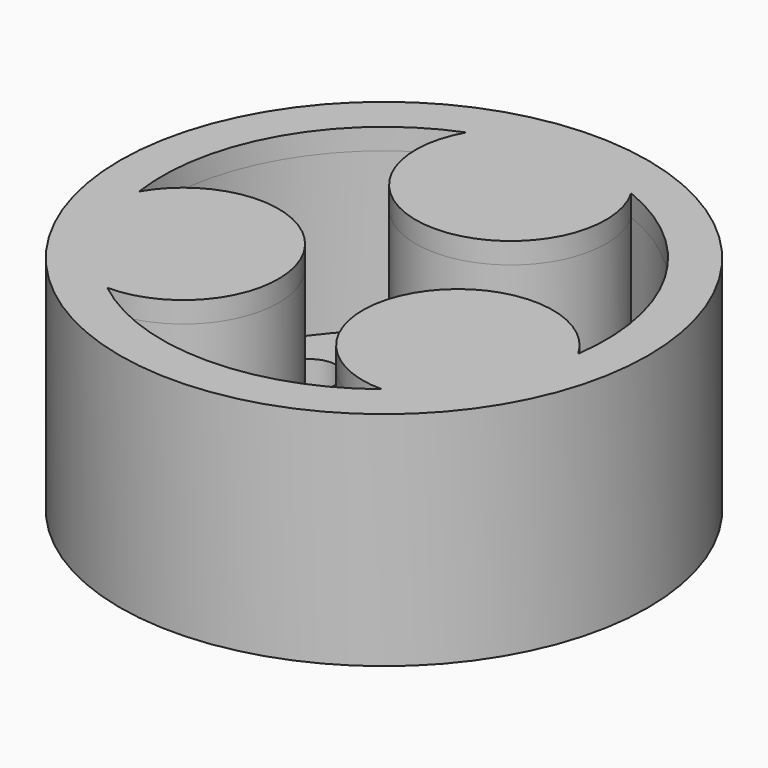
from build123d import *

# Parameters (mm, degrees)
F0_R     = 25
F0_R_2   = 5
F0_R_3   = 2.5
F0_R_4   = 3.5
F1_DEPTH = 19
F2_T     = -4
F3_DEPTH = 25
F4_R     = 25
F5_DEPTH = 2


# Not quite as in the source:
# - a feature names something its author has since deleted; it is built from what else it names


with BuildPart() as f1:
    # F0 (on Top) → F1 (new body)
    with BuildSketch(Plane.XY):
        Circle(F0_R)
        with Locations((-12.990381, -7.5)):
            Circle(F0_R_2, mode=Mode.SUBTRACT)
        with Locations((0, -15)):
            Circle(F0_R_3, mode=Mode.SUBTRACT)
        with Locations((12.990381, -7.5)):
            Circle(F0_R_2, mode=Mode.SUBTRACT)
        with Locations((-12.990381, 7.5)):
            Circle(F0_R_3, mode=Mode.SUBTRACT)
        Circle(F0_R_4, mode=Mode.SUBTRACT)
        with Locations((12.990381, 7.5)):
            Circle(F0_R_3, mode=Mode.SUBTRACT)
        with Locations((0, 15)):
            Circle(F0_R_2, mode=Mode.SUBTRACT)
        Circle(F0_R_4)
        with Locations((-12.990381, 7.5)):
            Circle(F0_R_3)
        with Locations((12.990381, 7.5)):
            Circle(F0_R_3)
        with Locations((0, -15)):
            Circle(F0_R_3)
    extrude(amount=F1_DEPTH)

    # F2
    f2_openings = [f1.faces().sort_by_distance(p)[0] for p in [
        (0, 0, 19),
    ]]
    offset(amount=F2_T, openings=f2_openings)

    # F0 (on Top) → F3 (cut)
    with BuildSketch(Plane.XY):
        with Locations((-12.990381, 7.5)):
            Circle(F0_R_3)
        Circle(F0_R_4)
        with Locations((12.990381, 7.5)):
            Circle(F0_R_3)
        with Locations((0, -15)):
            Circle(F0_R_3)
    extrude(amount=F3_DEPTH, mode=Mode.SUBTRACT)

    # F4 (on face) → F5 (join)
    with BuildSketch(Plane.XY.offset(19)):
        Circle(F4_R)
        with BuildLine():
            ThreePointArc((-20.78461, -3), (-18.186533, 10.5), (-7.794229, 19.5))
            ThreePointArc((-7.794229, 19.5), (0, 6), (7.794229, 19.5))
            ThreePointArc((7.794229, 19.5), (18.186533, 10.5), (20.78461, -3))
            ThreePointArc((20.78461, -3), (5.196152, -3), (12.990381, -16.5))
            ThreePointArc((12.990381, -16.5), (0, -21), (-12.990381, -16.5))
            ThreePointArc((-12.990381, -16.5), (-5.196152, -3), (-20.78461, -3))
        make_face(mode=Mode.SUBTRACT)
    extrude(amount=F5_DEPTH)


solid = f1.part
